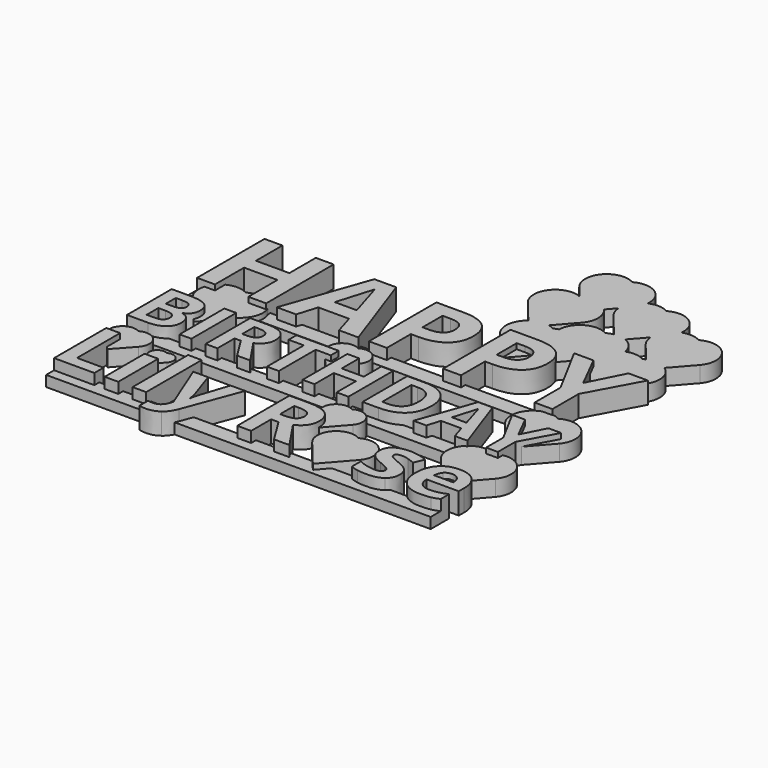
from build123d import *

# Parameters (mm, degrees)
F0_TEXT_SIZE   = 22.0588235294
F0_TEXT_SIZE_2 = 14.6296860713
F0_W           = 2.5421468203
F0_H           = 9.3203158344
F0_H_2         = 12.9721510883
F1_DEPTH       = 4
F2_W           = 69.2715635477
F2_H           = 3
F2_W_2         = 71.8336534358
F2_W_3         = 66.3625919118
F3_DEPTH       = 2
F5_DEPTH       = 3


# Not quite as in the source:
# - Text() gives the source's letters only with a copy of the font that has no kerning and outlines rounded to 1/6400 em; it was checked with that copy


with BuildPart() as f1:
    # F0 (on Top) → F1 (new body)
    with BuildSketch(Plane.XY):
        with Locations((-37.5, 11.5387746485)):
            Text('HAPPY', F0_TEXT_SIZE, font='Open Sans', font_style=FontStyle.BOLD, text_align=(TextAlign.LEFT, TextAlign.BOTTOM))
        with Locations((-37.5, -3.9945993228)):
            Text('BIRTHDAY', F0_TEXT_SIZE_2, font='Open Sans', font_style=FontStyle.BOLD, text_align=(TextAlign.LEFT, TextAlign.BOTTOM))
        Polygon((-35.9661758429, -9.0986326135), (-35.9661758429, -21.2865327415), (-28.4384336321, -21.2865327415), (-28.4384336321, -19.152516523), (-33.3813486983, -19.152516523), (-33.3813486983, -9.0986326135), align=None)
        with Locations((-25.2494131455, -16.6263748243)):
            Rectangle(F0_W, F0_H)
        with Locations((-20.0397460521, -14.8004571973)):
            Rectangle(F0_W, F0_H_2)
        with BuildLine():
            Line((-14.6500213402, -11.9662169071), (-17.4349125053, -11.9662169071))
            Line((-17.4349125053, -11.9662169071), (-13.7323943662, -21.2198447347))
            Line((-13.7323943662, -21.2198447347), (-13.8844430218, -21.6786582217))
            add(Edge.make_bspline(
                [(-14.6713615023, -22.9243901892), (-14.1672001707, -22.5109245469), (-13.8844430218, -21.6786582217)],
                knots=[0, 0, 0, 1, 1, 1], degree=2))
            add(Edge.make_bspline(
                [(-15.8504054631, -23.3378558316), (-15.175522834, -23.3378558316), (-14.6713615023, -22.9243901892)],
                knots=[0, 0, 0, 1, 1, 1], degree=2))
            add(Edge.make_bspline(
                [(-16.8507255655, -23.2284875004), (-16.3919120785, -23.3378558316), (-15.8504054631, -23.3378558316)],
                knots=[0, 0, 0, 1, 1, 1], degree=2))
            Line((-16.8507255655, -23.2284875004), (-16.8507255655, -25.2451328269))
            add(Edge.make_bspline(
                [(-15.5596457533, -25.3891789216), (-16.2185232608, -25.3891789216), (-16.8507255655, -25.2451328269)],
                knots=[0, 0, 0, 1, 1, 1], degree=2))
            add(Edge.make_bspline(
                [(-13.2135616731, -24.6636134073), (-14.2178830559, -25.3891789216), (-15.5596457533, -25.3891789216)],
                knots=[0, 0, 0, 1, 1, 1], degree=2))
            add(Edge.make_bspline(
                [(-11.6650661545, -22.4789143036), (-12.2092402902, -23.938047893), (-13.2135616731, -24.6636134073)],
                knots=[0, 0, 0, 1, 1, 1], degree=2))
            Line((-11.6650661545, -22.4789143036), (-7.7224711908, -11.9662169071))
            Line((-7.7224711908, -11.9662169071), (-10.4486769099, -11.9662169071))
            Line((-10.4486769099, -11.9662169071), (-12.1745625267, -17.2105617641))
            add(Edge.make_bspline(
                [(-12.5320102433, -18.8270790497), (-12.441314554, -17.9681375217), (-12.1745625267, -17.2105617641)],
                knots=[0, 0, 0, 1, 1, 1], degree=2))
            Line((-12.5320102433, -18.8270790497), (-12.5826931285, -18.8270790497))
            add(Edge.make_bspline(
                [(-12.8921254802, -17.2105617641), (-12.6653862569, -17.8934469541), (-12.5826931285, -18.8270790497)],
                knots=[0, 0, 0, 1, 1, 1], degree=2))
            Line((-12.8921254802, -17.2105617641), (-14.6500213402, -11.9662169071))
        make_face()
        with BuildLine():
            Line((0.8322663252, -21.2865327415), (0.8322663252, -16.6103697027))
            Line((0.8322663252, -16.6103697027), (2.2060392659, -16.6103697027))
            Line((2.2060392659, -16.6103697027), (5.1163038839, -21.2865327415))
            Line((5.1163038839, -21.2865327415), (7.9838881776, -21.2865327415))
            add(Edge.make_bspline(
                [(4.3987409304, -15.9754998777), (7.1516218523, -20.0861486186), (7.9838881776, -21.2865327415)],
                knots=[0, 0, 0, 1, 1, 1], degree=2))
            add(Edge.make_bspline(
                [(6.0752774221, -14.6630799033), (5.4844216816, -15.5006812691), (4.3987409304, -15.9754998777)],
                knots=[0, 0, 0, 1, 1, 1], degree=2))
            add(Edge.make_bspline(
                [(6.6661331626, -12.7504678674), (6.6661331626, -13.8254785375), (6.0752774221, -14.6630799033)],
                knots=[0, 0, 0, 1, 1, 1], degree=2))
            add(Edge.make_bspline(
                [(5.4750853606, -10.0029219861), (6.6661331626, -10.9072113587), (6.6661331626, -12.7504678674)],
                knots=[0, 0, 0, 1, 1, 1], degree=2))
            add(Edge.make_bspline(
                [(1.7979086641, -9.0986326135), (4.2840375587, -9.0986326135), (5.4750853606, -10.0029219861)],
                knots=[0, 0, 0, 1, 1, 1], degree=2))
            Line((1.7979086641, -9.0986326135), (-1.7525608195, -9.0986326135))
            Line((-1.7525608195, -9.0986326135), (-1.7525608195, -21.2865327415))
            Line((-1.7525608195, -21.2865327415), (0.8322663252, -21.2865327415))
        make_face()
        with BuildLine():
            Line((1.6645326504, -14.5083637274), (0.8322663252, -14.5083637274))
            Line((0.8322663252, -14.5083637274), (0.8322663252, -11.2166437104))
            Line((0.8322663252, -11.2166437104), (1.6165172855, -11.2166437104))
            add(Edge.make_bspline(
                [(3.4611075544, -11.5834277479), (2.8649167734, -11.2166437104), (1.6165172855, -11.2166437104)],
                knots=[0, 0, 0, 1, 1, 1], degree=2))
            add(Edge.make_bspline(
                [(4.0572983355, -12.8171558743), (4.0572983355, -11.9502117855), (3.4611075544, -11.5834277479)],
                knots=[0, 0, 0, 1, 1, 1], degree=2))
            add(Edge.make_bspline(
                [(3.4744451558, -14.1002331256), (4.0572983355, -13.6921025239), (4.0572983355, -12.8171558743)],
                knots=[0, 0, 0, 1, 1, 1], degree=2))
            add(Edge.make_bspline(
                [(1.6645326504, -14.5083637274), (2.8915919761, -14.5083637274), (3.4744451558, -14.1002331256)],
                knots=[0, 0, 0, 1, 1, 1], degree=2))
        make_face(mode=Mode.SUBTRACT)
        with BuildLine():
            add(Edge.make_bspline(
                [(26.3924455826, -18.517646698), (26.3924455826, -19.9527726049), (25.3961267606, -20.7036795618)],
                knots=[0, 0, 0, 1, 1, 1], degree=2))
            add(Edge.make_bspline(
                [(26.1497012377, -17.326598896), (26.3924455826, -17.8267589472), (26.3924455826, -18.517646698)],
                knots=[0, 0, 0, 1, 1, 1], degree=2))
            add(Edge.make_bspline(
                [(25.3987942808, -16.4436496856), (25.9069568929, -16.8264388448), (26.1497012377, -17.326598896)],
                knots=[0, 0, 0, 1, 1, 1], degree=2))
            add(Edge.make_bspline(
                [(23.7996158771, -15.6180521611), (24.8906316688, -16.0608605264), (25.3987942808, -16.4436496856)],
                knots=[0, 0, 0, 1, 1, 1], degree=2))
            add(Edge.make_bspline(
                [(22.2097737943, -14.8764815251), (22.5725565514, -15.1272284308), (23.7996158771, -15.6180521611)],
                knots=[0, 0, 0, 1, 1, 1], degree=2))
            add(Edge.make_bspline(
                [(21.8469910371, -14.2842920245), (21.8469910371, -14.6257346195), (22.2097737943, -14.8764815251)],
                knots=[0, 0, 0, 1, 1, 1], degree=2))
            add(Edge.make_bspline(
                [(22.9726845924, -13.6760974022), (21.8469910371, -13.6760974022), (21.8469910371, -14.2842920245)],
                knots=[0, 0, 0, 1, 1, 1], degree=2))
            add(Edge.make_bspline(
                [(24.2157490397, -13.8681588619), (23.6075544174, -13.6760974022), (22.9726845924, -13.6760974022)],
                knots=[0, 0, 0, 1, 1, 1], degree=2))
            add(Edge.make_bspline(
                [(25.5255014938, -14.3589825921), (24.823943662, -14.0602203215), (24.2157490397, -13.8681588619)],
                knots=[0, 0, 0, 1, 1, 1], degree=2))
            Line((25.5255014938, -14.3589825921), (26.2910798122, -12.5263961645))
            add(Edge.make_bspline(
                [(23.0153649168, -11.7928280894), (24.6985702091, -11.7928280894), (26.2910798122, -12.5263961645)],
                knots=[0, 0, 0, 1, 1, 1], degree=2))
            add(Edge.make_bspline(
                [(20.2851579172, -12.4717119989), (21.2467989757, -11.7928280894), (23.0153649168, -11.7928280894)],
                knots=[0, 0, 0, 1, 1, 1], degree=2))
            add(Edge.make_bspline(
                [(19.3235168587, -14.3936603557), (19.3235168587, -13.1505959084), (20.2851579172, -12.4717119989)],
                knots=[0, 0, 0, 1, 1, 1], degree=2))
            add(Edge.make_bspline(
                [(19.5515898421, -15.6127171205), (19.3235168587, -15.1165583497), (19.3235168587, -14.3936603557)],
                knots=[0, 0, 0, 1, 1, 1], degree=2))
            add(Edge.make_bspline(
                [(20.2851579172, -16.4929988107), (19.7796628254, -16.1088758913), (19.5515898421, -15.6127171205)],
                knots=[0, 0, 0, 1, 1, 1], degree=2))
            add(Edge.make_bspline(
                [(21.865663679, -17.3279326562), (20.790653009, -16.87712173), (20.2851579172, -16.4929988107)],
                knots=[0, 0, 0, 1, 1, 1], degree=2))
            add(Edge.make_bspline(
                [(23.0647140418, -17.8801093527), (22.6152368758, -17.6427000484), (21.865663679, -17.3279326562)],
                knots=[0, 0, 0, 1, 1, 1], degree=2))
            add(Edge.make_bspline(
                [(23.6982501067, -18.3055788363), (23.5141912079, -18.117518657), (23.0647140418, -17.8801093527)],
                knots=[0, 0, 0, 1, 1, 1], degree=2))
            add(Edge.make_bspline(
                [(23.8823090055, -18.7950688064), (23.8823090055, -18.4936390155), (23.6982501067, -18.3055788363)],
                knots=[0, 0, 0, 1, 1, 1], degree=2))
            add(Edge.make_bspline(
                [(22.4978659838, -19.5953248883), (23.8823090055, -19.5953248883), (23.8823090055, -18.7950688064)],
                knots=[0, 0, 0, 1, 1, 1], degree=2))
            add(Edge.make_bspline(
                [(20.9346991037, -19.3699194253), (21.8229833547, -19.5953248883), (22.4978659838, -19.5953248883)],
                knots=[0, 0, 0, 1, 1, 1], degree=2))
            add(Edge.make_bspline(
                [(19.3395219804, -18.811073928), (20.0464148528, -19.1445139622), (20.9346991037, -19.3699194253)],
                knots=[0, 0, 0, 1, 1, 1], degree=2))
            Line((19.3395219804, -18.811073928), (19.3395219804, -20.910412383))
            add(Edge.make_bspline(
                [(20.6812846778, -21.3158754645), (19.9637217243, -21.1771644103), (19.3395219804, -20.910412383)],
                knots=[0, 0, 0, 1, 1, 1], degree=2))
            add(Edge.make_bspline(
                [(22.4151728553, -21.4545865187), (21.3988476312, -21.4545865187), (20.6812846778, -21.3158754645)],
                knots=[0, 0, 0, 1, 1, 1], degree=2))
            add(Edge.make_bspline(
                [(25.3961267606, -20.7036795618), (24.3998079385, -21.4545865187), (22.4151728553, -21.4545865187)],
                knots=[0, 0, 0, 1, 1, 1], degree=2))
        make_face()
        with BuildLine():
            add(Edge.make_bspline(
                [(32.5917626974, -21.4545865187), (30.3430431071, -21.4545865187), (29.0759709774, -20.2115220714)],
                knots=[0, 0, 0, 1, 1, 1], degree=2))
            add(Edge.make_bspline(
                [(34.443021767, -21.2918677821), (33.6854460094, -21.4545865187), (32.5917626974, -21.4545865187)],
                knots=[0, 0, 0, 1, 1, 1], degree=2))
            add(Edge.make_bspline(
                [(35.8674775928, -20.7957090113), (35.2005975245, -21.1291490454), (34.443021767, -21.2918677821)],
                knots=[0, 0, 0, 1, 1, 1], degree=2))
            Line((35.8674775928, -20.7957090113), (35.8674775928, -18.8270790497))
            add(Edge.make_bspline(
                [(34.3016431925, -19.3859245469), (35.0512163892, -19.211201969), (35.8674775928, -18.8270790497)],
                knots=[0, 0, 0, 1, 1, 1], degree=2))
            add(Edge.make_bspline(
                [(32.7091335894, -19.5606471248), (33.5520699957, -19.5606471248), (34.3016431925, -19.3859245469)],
                knots=[0, 0, 0, 1, 1, 1], degree=2))
            add(Edge.make_bspline(
                [(31.0259282971, -18.9524525025), (31.6261203585, -19.5606471248), (32.7091335894, -19.5606471248)],
                knots=[0, 0, 0, 1, 1, 1], degree=2))
            add(Edge.make_bspline(
                [(30.3830559112, -17.2612446493), (30.4257362356, -18.3442578802), (31.0259282971, -18.9524525025)],
                knots=[0, 0, 0, 1, 1, 1], degree=2))
            Line((30.3830559112, -17.2612446493), (36.3929790866, -17.2612446493))
            Line((36.3929790866, -17.2612446493), (36.3929790866, -16.0261827629))
            add(Edge.make_bspline(
                [(35.292626974, -12.9171878845), (36.3929790866, -14.0415476796), (36.3929790866, -16.0261827629)],
                knots=[0, 0, 0, 1, 1, 1], degree=2))
            add(Edge.make_bspline(
                [(32.2183098592, -11.7928280894), (34.1922748613, -11.7928280894), (35.292626974, -12.9171878845)],
                knots=[0, 0, 0, 1, 1, 1], degree=2))
            add(Edge.make_bspline(
                [(28.9799402475, -13.0719040603), (30.1509816475, -11.7928280894), (32.2183098592, -11.7928280894)],
                knots=[0, 0, 0, 1, 1, 1], degree=2))
            add(Edge.make_bspline(
                [(27.8088988476, -16.6930628312), (27.8088988476, -14.3509800313), (28.9799402475, -13.0719040603)],
                knots=[0, 0, 0, 1, 1, 1], degree=2))
            add(Edge.make_bspline(
                [(29.0759709774, -20.2115220714), (27.8088988476, -18.9684576242), (27.8088988476, -16.6930628312)],
                knots=[0, 0, 0, 1, 1, 1], degree=2))
        make_face()
        with BuildLine():
            add(Edge.make_bspline(
                [(32.2343149808, -13.6014068346), (31.426056338, -13.6014068346), (30.967242851, -14.113570727)],
                knots=[0, 0, 0, 1, 1, 1], degree=2))
            add(Edge.make_bspline(
                [(33.5173922322, -14.113570727), (33.0425736236, -13.6014068346), (32.2343149808, -13.6014068346)],
                knots=[0, 0, 0, 1, 1, 1], degree=2))
            add(Edge.make_bspline(
                [(34.0108834827, -15.5673692759), (33.9922108408, -14.6257346195), (33.5173922322, -14.113570727)],
                knots=[0, 0, 0, 1, 1, 1], degree=2))
            Line((34.0108834827, -15.5673692759), (30.4417413572, -15.5673692759))
            add(Edge.make_bspline(
                [(30.967242851, -14.113570727), (30.5084293641, -14.6257346195), (30.4417413572, -15.5673692759)],
                knots=[0, 0, 0, 1, 1, 1], degree=2))
        make_face(mode=Mode.SUBTRACT)
    extrude(amount=F1_DEPTH)

    # F2 (on Top) → F3 (join)
    with BuildSketch(Plane.XY):
        with Locations((-1.5498323682, -4.4945993228)):
            Rectangle(F2_W, F2_H)
        with Locations((-0.0493491251, -21.652516523)):
            Rectangle(F2_W_2, F2_H)
        with Locations((-2.3368566176, 11.0387746485)):
            Rectangle(F2_W_3, F2_H)
    extrude(amount=F3_DEPTH)

    # F4 (on Top) → F5 (join)
    with BuildSketch(Plane.XY):
        with BuildLine():
            ThreePointArc((15.8710453597, 42.3152042751), (13.5240060481, 43.5901863002), (10.8977104083, 43.1036229369))
            ThreePointArc((10.8977104083, 43.1036229369), (10.6969632271, 43.2120119507), (10.4903631205, 43.3087797398))
            Line((10.4903631205, 43.3087797398), (13.5120771973, 39.6303699124))
            Line((13.5120771973, 39.6303699124), (15.8710453597, 42.3152042751))
        make_face()
        with BuildLine():
            ThreePointArc((10.4903631205, 43.3087797398), (10.6969632271, 43.2120119507), (10.8977104083, 43.1036229369))
            ThreePointArc((10.8977104083, 43.1036229369), (13.5240060481, 43.5901863002), (15.8710453597, 42.3152042751))
            Line((15.8710453597, 42.3152042751), (17.28911835, 43.9291688694))
            ThreePointArc((17.28911835, 43.9291688694), (17.8752784968, 46.2349552383), (19.667146129, 47.8000254877))
            ThreePointArc((19.667146129, 47.8000254877), (17.8364951333, 51.5292442561), (13.6832215476, 51.6223797092))
            ThreePointArc((13.6832215476, 51.6223797092), (8.632499056, 50.7453792284), (8.5923837689, 45.6192385462))
            Line((8.5923837689, 45.6192385462), (10.4903631205, 43.3087797398))
        make_face()
        with BuildLine():
            Line((13.5120771973, 39.6303699124), (10.4903631205, 43.3087797398))
            ThreePointArc((10.4903631205, 43.3087797398), (5.7044549328, 42.0484877948), (5.8068726296, 37.1004817739))
            Line((5.8068726296, 37.1004817739), (9.434985023, 32.6838877668))
            ThreePointArc((9.434985023, 32.6838877668), (11.0020288677, 33.3963663052), (12.7233963769, 33.3842841927))
            Line((12.7233963769, 33.3842841927), (15.988548187, 37.1004817739))
            ThreePointArc((15.988548187, 37.1004817739), (16.8966953315, 39.7296300543), (15.8710453597, 42.3152042751))
            Line((15.8710453597, 42.3152042751), (13.5120771973, 39.6303699124))
        make_face()
        with BuildLine():
            Line((18.7740593263, 45.6192385462), (17.28911835, 43.9291688694))
            ThreePointArc((17.28911835, 43.9291688694), (17.5547067733, 42.6933470485), (18.1926598963, 41.6021052805))
            Line((18.1926598963, 41.6021052805), (21.9117701176, 37.0747372903))
            ThreePointArc((21.9117701176, 37.0747372903), (23.0705080697, 37.1278805872), (24.1957729049, 36.8463190445))
            Line((24.1957729049, 36.8463190445), (26.6866230167, 39.6812534361))
            ThreePointArc((26.6866230167, 39.6812534361), (27.3192394754, 42.0896780932), (29.2541092545, 43.6571575508))
            ThreePointArc((29.2541092545, 43.6571575508), (27.4897793831, 47.4776581319), (23.2834976751, 47.6052464435))
            ThreePointArc((23.2834976751, 47.6052464435), (21.4986284564, 48.1353554822), (19.667146129, 47.8000254877))
            ThreePointArc((19.667146129, 47.8000254877), (19.3848459929, 46.6423702915), (18.7740593263, 45.6192385462))
        make_face()
        with BuildLine():
            ThreePointArc((19.667146129, 47.8000254877), (17.8752784968, 46.2349552383), (17.28911835, 43.9291688694))
            Line((17.28911835, 43.9291688694), (18.7740593263, 45.6192385462))
            ThreePointArc((18.7740593263, 45.6192385462), (19.3848459929, 46.6423702915), (19.667146129, 47.8000254877))
        make_face()
        with BuildLine():
            ThreePointArc((12.7233963769, 33.3842841927), (11.0020288677, 33.3963663052), (9.434985023, 32.6838877668))
            Line((9.434985023, 32.6838877668), (10.726566058, 31.1116131401))
            Line((10.726566058, 31.1116131401), (12.7233963769, 33.3842841927))
        make_face()
        with BuildLine():
            Line((10.726566058, 31.1116131401), (9.434985023, 32.6838877668))
            ThreePointArc((9.434985023, 32.6838877668), (7.8639413359, 29.961977531), (8.7444575695, 26.9450809863))
            Line((8.7444575695, 26.9450809863), (13.6641509979, 20.9562123525))
            Line((13.6641509979, 20.9562123525), (18.7530286138, 26.7480639377))
            Line((18.7530286138, 26.7480639377), (15.5816244153, 30.6086953786))
            ThreePointArc((15.5816244153, 30.6086953786), (14.8796431709, 31.877095773), (14.6758527891, 33.3123959883))
            ThreePointArc((14.6758527891, 33.3123959883), (14.2451145511, 33.1544509053), (13.8352953482, 32.9482221494))
            ThreePointArc((13.8352953482, 32.9482221494), (13.2957128961, 33.2079868833), (12.7233963769, 33.3842841927))
            Line((12.7233963769, 33.3842841927), (10.726566058, 31.1116131401))
        make_face()
        with BuildLine():
            Line((23.1123533248, 35.6132366467), (21.9117701176, 37.0747372903))
            ThreePointArc((21.9117701176, 37.0747372903), (21.2728463678, 36.8948772429), (20.672462194, 36.6118365416))
            ThreePointArc((20.672462194, 36.6118365416), (16.7442015088, 36.6522763701), (14.6758527891, 33.3123959883))
            ThreePointArc((14.6758527891, 33.3123959883), (19.1621928454, 31.7048755956), (18.9261331269, 26.9450809863))
            Line((18.9261331269, 26.9450809863), (18.7530286138, 26.7480639377))
            Line((18.7530286138, 26.7480639377), (20.5013178437, 24.6198267448))
            Line((20.5013178437, 24.6198267448), (24.2263502902, 28.8594325496))
            ThreePointArc((24.2263502902, 28.8594325496), (24.4135741152, 31.8368320124), (26.6091530057, 33.8565829024))
            ThreePointArc((26.6091530057, 33.8565829024), (25.7849426689, 35.6601969249), (24.1957729049, 36.8463190445))
            Line((24.1957729049, 36.8463190445), (23.1123533248, 35.6132366467))
        make_face()
        with BuildLine():
            ThreePointArc((18.9261331269, 26.9450809863), (19.1621928454, 31.7048755956), (14.6758527891, 33.3123959883))
            ThreePointArc((14.6758527891, 33.3123959883), (14.8796431709, 31.877095773), (15.5816244153, 30.6086953786))
            Line((15.5816244153, 30.6086953786), (18.7530286138, 26.7480639377))
            Line((18.7530286138, 26.7480639377), (18.9261331269, 26.9450809863))
        make_face()
        with BuildLine():
            ThreePointArc((28.3743354538, 41.6021052805), (28.9607013297, 42.566923344), (29.2541092545, 43.6571575508))
            ThreePointArc((29.2541092545, 43.6571575508), (27.3192394754, 42.0896780932), (26.6866230167, 39.6812534361))
            Line((26.6866230167, 39.6812534361), (28.3743354538, 41.6021052805))
        make_face()
        with BuildLine():
            ThreePointArc((32.6795068222, 43.3838480601), (30.9976522422, 43.9070743086), (29.2541092545, 43.6571575508))
            ThreePointArc((29.2541092545, 43.6571575508), (28.9607013297, 42.566923344), (28.3743354538, 41.6021052805))
            Line((28.3743354538, 41.6021052805), (26.6866230167, 39.6812534361))
            ThreePointArc((26.6866230167, 39.6812534361), (26.9555430113, 38.4595774361), (27.5886690435, 37.3807068971))
            Line((27.5886690435, 37.3807068971), (30.5142626527, 33.8193069732))
            ThreePointArc((30.5142626527, 33.8193069732), (32.4509480968, 34.0923705397), (34.2855856515, 33.414565801))
            Line((34.2855856515, 33.414565801), (37.7703446009, 37.3807068971))
            ThreePointArc((37.7703446009, 37.3807068971), (37.7302293138, 42.5068475793), (32.6795068222, 43.3838480601))
        make_face()
        with BuildLine():
            ThreePointArc((30.0241161722, 33.5793105403), (28.347824397, 34.1020890319), (26.6091530057, 33.8565829024))
            ThreePointArc((26.6091530057, 33.8565829024), (26.5433448923, 32.1396341697), (25.7632999727, 30.6086953786))
            Line((25.7632999727, 30.6086953786), (24.2263502902, 28.8594325496))
            ThreePointArc((24.2263502902, 28.8594325496), (24.5205599516, 28.1851587162), (24.9332783935, 27.5761693773))
            Line((24.9332783935, 27.5761693773), (29.8529718219, 21.5873007435))
            Line((29.8529718219, 21.5873007435), (34.9397683559, 27.3767837676))
            ThreePointArc((34.9397683559, 27.3767837676), (36.0008422313, 30.5460799625), (34.2855856515, 33.414565801))
            Line((34.2855856515, 33.414565801), (32.508362472, 31.3918382633))
            Line((32.508362472, 31.3918382633), (30.5142626527, 33.8193069732))
            ThreePointArc((30.5142626527, 33.8193069732), (30.2650915834, 33.7076777832), (30.0241161722, 33.5793105403))
        make_face()
        with BuildLine():
            ThreePointArc((25.7632999727, 30.6086953786), (26.5433448923, 32.1396341697), (26.6091530057, 33.8565829024))
            ThreePointArc((26.6091530057, 33.8565829024), (24.4135741152, 31.8368320124), (24.2263502902, 28.8594325496))
            Line((24.2263502902, 28.8594325496), (25.7632999727, 30.6086953786))
        make_face()
        with BuildLine():
            Line((32.508362472, 31.3918382633), (34.2855856515, 33.414565801))
            ThreePointArc((34.2855856515, 33.414565801), (32.4509480968, 34.0923705397), (30.5142626527, 33.8193069732))
            Line((30.5142626527, 33.8193069732), (32.508362472, 31.3918382633))
        make_face()
        with BuildLine():
            ThreePointArc((-23.460767245, -10.5974629963), (-23.3785588051, -8.6388796142), (-25.3041368139, -8.2715154565))
            ThreePointArc((-25.3041368139, -8.2715154565), (-27.1981577482, -8.6003906368), (-27.2132009809, -10.5226933926))
            Line((-27.2132009809, -10.5226933926), (-25.3683159452, -12.7685191303))
            Line((-25.3683159452, -12.7685191303), (-23.460767245, -10.5974629963))
        make_face()
        with BuildLine():
            ThreePointArc((17.7506930834, -17.0362158441), (17.7155922072, -12.5508427471), (13.296210027, -11.7834673264))
            ThreePointArc((13.296210027, -11.7834673264), (8.8768278469, -12.5508427471), (8.8417269707, -17.0362158441))
            Line((8.8417269707, -17.0362158441), (13.1464587205, -22.2764758987))
            Line((13.1464587205, -22.2764758987), (17.7506930834, -17.0362158441))
        make_face()
        with BuildLine():
            ThreePointArc((37.2771124401, 5.1807187554), (37.236997153, 10.3068594377), (32.1862746614, 11.1838599185))
            ThreePointArc((32.1862746614, 11.1838599185), (27.1355521698, 10.3068594377), (27.0954368827, 5.1807187554))
            Line((27.0954368827, 5.1807187554), (32.0151303111, -0.8081498784))
            Line((32.0151303111, -0.8081498784), (37.2771124401, 5.1807187554))
        make_face()
        with BuildLine():
            ThreePointArc((-23.3789527746, 7.6379913258), (-23.1597302683, 12.8608803447), (-28.2946049583, 13.8405180985))
            ThreePointArc((-28.2946049583, 13.8405180985), (-33.3453274499, 12.9635176177), (-33.385442737, 7.8373769355))
            Line((-33.385442737, 7.8373769355), (-28.4657493086, 1.8485083017))
            Line((-28.4657493086, 1.8485083017), (-23.3789527746, 7.6379913258))
        make_face()
        with BuildLine():
            ThreePointArc((36.8976171174, -9.3308138604), (36.8575018303, -4.2046731782), (31.8067793387, -3.3276726974))
            ThreePointArc((31.8067793387, -3.3276726974), (26.7560568471, -4.2046731782), (26.71594156, -9.3308138604))
            Line((26.71594156, -9.3308138604), (31.6356349884, -15.3196824942))
            Line((31.6356349884, -15.3196824942), (36.8976171174, -9.3308138604))
        make_face()
        with BuildLine():
            ThreePointArc((-29.7967798697, -9.3315176463), (-29.6597658033, -6.0672120096), (-32.8690624845, -5.4549384134))
            ThreePointArc((-32.8690624845, -5.4549384134), (-36.0630556223, -6.0480952208), (-35.9745223626, -9.2954924901))
            Line((-35.9745223626, -9.2954924901), (-32.8690624845, -12.7345188382))
            Line((-32.8690624845, -12.7345188382), (-29.7967798697, -9.3315176463))
        make_face()
        with BuildLine():
            ThreePointArc((-1.4179188738, 6.4611722219), (-1.2809048074, 9.7254778587), (-4.4902014886, 10.3377514548))
            ThreePointArc((-4.4902014886, 10.3377514548), (-7.6469030459, 9.7896261543), (-7.6719751003, 6.5857882279))
            Line((-7.6719751003, 6.5857882279), (-4.5971667076, 2.8427453318))
            Line((-4.5971667076, 2.8427453318), (-1.4179188738, 6.4611722219))
        make_face()
        with BuildLine():
            ThreePointArc((10.0142014591, -9.0243846608), (9.9891294046, -5.8205467344), (6.8324278474, -5.2724214339))
            ThreePointArc((6.8324278474, -5.2724214339), (3.6757262901, -5.8205467344), (3.6506542357, -9.0243846608))
            Line((3.6506542357, -9.0243846608), (6.7254626285, -12.7674275569))
            Line((6.7254626285, -12.7674275569), (10.0142014591, -9.0243846608))
        make_face()
        with BuildLine():
            ThreePointArc((24.1957729049, 36.8463190445), (23.0705080697, 37.1278805872), (21.9117701176, 37.0747372903))
            Line((21.9117701176, 37.0747372903), (23.1123533248, 35.6132366467))
            Line((23.1123533248, 35.6132366467), (24.1957729049, 36.8463190445))
        make_face()
    extrude(amount=F5_DEPTH)


solid = f1.part
